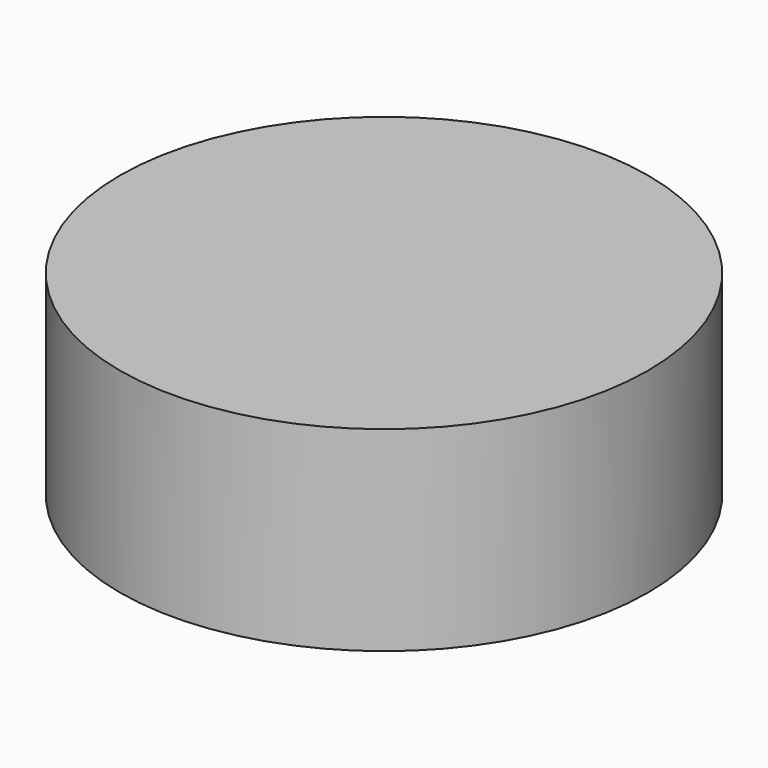
from build123d import *

# Parameters (mm, degrees)
F5_R     = 3.4326019605
F6_DEPTH = 2.54


# Not quite as in the source:
# - a feature of the source that left no trace in its solid (it failed there, or was rolled back) is left out
# - the program builds the solid bodies; features that only make, move or delete a surface that nothing else refers to are left out


with BuildPart() as f6:
    # F5 (on offset) → F6 (new body)
    with BuildSketch(Plane.XY.offset(25.4)):
        with Locations((0, 17.0013140887)):
            Circle(F5_R)
    extrude(amount=-F6_DEPTH)


solid = f6.part
